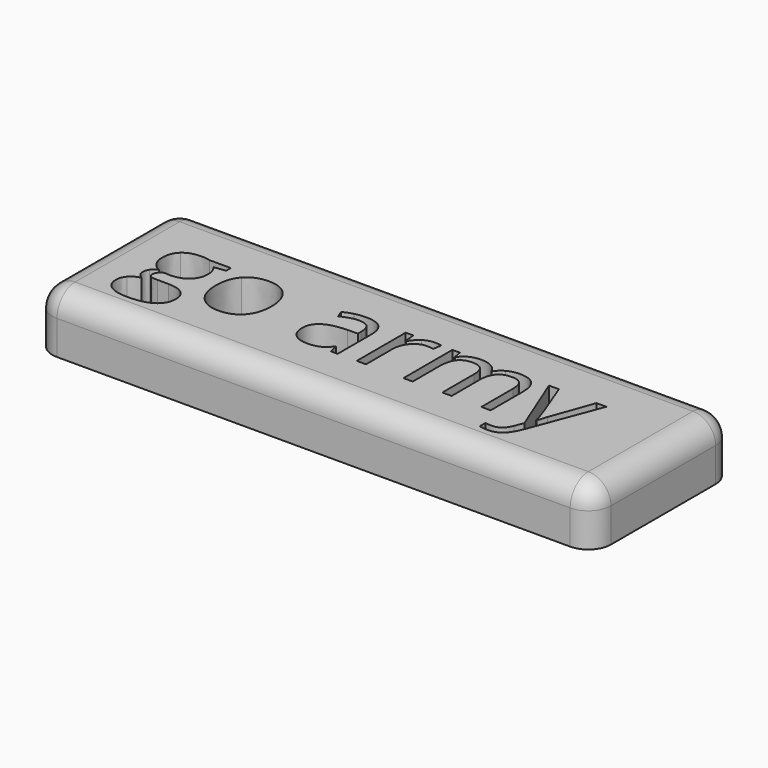
from build123d import *

# Parameters (mm, degrees)
F0_W         = 124.970305711
F0_H         = 39.4006967545
F1_DEPTH     = 12.7
F2_R         = 5.08
F3_T1_DEPTH  = 20.32
F3_S5_W      = 5.08
F3_S5_H      = 5.08
F3_T6_DEPTH  = 5.08
F3_S11_W     = 5.08
F3_S11_H     = 5.08
F3_T12_DEPTH = 5.08
F3_S17_W     = 5.08
F3_S17_H     = 5.08
F3_T18_DEPTH = 5.08
F3_S23_W     = 5.08
F3_S23_H     = 5.08
F3_T24_DEPTH = 5.08


# Not quite as in the source:
# - a fillet or chamfer that OpenCascade refuses, or shapes differently, is made with other operations: its cross-section is extruded or revolved along the edge and cut away or added


with BuildPart() as f1:
    # F0 (on Top) → F1 (new body)
    with BuildSketch(Plane.XY):
        with Locations((2.1755006164, 19.7003483772)):
            Rectangle(F0_W, F0_H)
        with BuildLine():
            Line((-42.0411116502, 26.2190565667), (-37.310148709, 26.2190565667))
            Line((-37.310148709, 26.2190565667), (-37.310148709, 24.9084519682))
            Line((-37.310148709, 24.9084519682), (-39.8434515001, 24.6087710386))
            add(Edge.make_bspline(
                [(-39.8434515001, 24.6087710386), (-39.4958216218, 24.1732347543), (-39.2201151666, 23.4659877606)],
                knots=[0, 0, 0, 1, 1, 1], degree=2))
            add(Edge.make_bspline(
                [(-39.2201151666, 23.4659877606), (-38.9444087115, 22.7587407668), (-38.9444087115, 21.8756809611)],
                knots=[0, 0, 0, 1, 1, 1], degree=2))
            add(Edge.make_bspline(
                [(-38.9444087115, 21.8756809611), (-38.9444087115, 19.8618251145), (-40.3189452417, 18.6631013963)],
                knots=[0, 0, 0, 1, 1, 1], degree=2))
            add(Edge.make_bspline(
                [(-40.3189452417, 18.6631013963), (-41.6934817719, 17.4643776781), (-44.0909292083, 17.4643776781)],
                knots=[0, 0, 0, 1, 1, 1], degree=2))
            add(Edge.make_bspline(
                [(-44.0909292083, 17.4643776781), (-44.7022783046, 17.4643776781), (-45.2377082321, 17.5642713212)],
                knots=[0, 0, 0, 1, 1, 1], degree=2))
            add(Edge.make_bspline(
                [(-45.2377082321, 17.5642713212), (-46.5603000678, 16.8650158189), (-46.5603000678, 15.8061432012)],
                knots=[0, 0, 0, 1, 1, 1], degree=2))
            add(Edge.make_bspline(
                [(-46.5603000678, 15.8061432012), (-46.5603000678, 15.2427430536), (-46.0987914363, 14.9750280899)],
                knots=[0, 0, 0, 1, 1, 1], degree=2))
            add(Edge.make_bspline(
                [(-46.0987914363, 14.9750280899), (-45.6372828048, 14.7073131262), (-44.5144782554, 14.7073131262)],
                knots=[0, 0, 0, 1, 1, 1], degree=2))
            Line((-44.5144782554, 14.7073131262), (-42.0930563446, 14.7073131262))
            add(Edge.make_bspline(
                [(-42.0930563446, 14.7073131262), (-39.8674259745, 14.7073131262), (-38.6766937477, 13.7703107531)],
                knots=[0, 0, 0, 1, 1, 1], degree=2))
            add(Edge.make_bspline(
                [(-38.6766937477, 13.7703107531), (-37.485961521, 12.83330838), (-37.485961521, 11.0472100399)],
                knots=[0, 0, 0, 1, 1, 1], degree=2))
            add(Edge.make_bspline(
                [(-37.485961521, 11.0472100399), (-37.485961521, 8.773630721), (-39.3080215727, 7.5809006214)],
                knots=[0, 0, 0, 1, 1, 1], degree=2))
            add(Edge.make_bspline(
                [(-39.3080215727, 7.5809006214), (-41.1300816243, 6.3881705218), (-44.6263591358, 6.3881705218)],
                knots=[0, 0, 0, 1, 1, 1], degree=2))
            add(Edge.make_bspline(
                [(-44.6263591358, 6.3881705218), (-47.3115002646, 6.3881705218), (-48.7659517094, 7.3871069536)],
                knots=[0, 0, 0, 1, 1, 1], degree=2))
            add(Edge.make_bspline(
                [(-48.7659517094, 7.3871069536), (-50.2204031541, 8.3860433854), (-50.2204031541, 10.2120991829)],
                knots=[0, 0, 0, 1, 1, 1], degree=2))
            add(Edge.make_bspline(
                [(-50.2204031541, 10.2120991829), (-50.2204031541, 11.4587718498), (-49.4212540086, 12.3717997485)],
                knots=[0, 0, 0, 1, 1, 1], degree=2))
            add(Edge.make_bspline(
                [(-49.4212540086, 12.3717997485), (-48.6221048632, 13.2848276472), (-47.1756449099, 13.6084830511)],
                knots=[0, 0, 0, 1, 1, 1], degree=2))
            add(Edge.make_bspline(
                [(-47.1756449099, 13.6084830511), (-47.6990876001, 13.844232049), (-48.0547089699, 14.343700265)],
                knots=[0, 0, 0, 1, 1, 1], degree=2))
            add(Edge.make_bspline(
                [(-48.0547089699, 14.343700265), (-48.4103303396, 14.8431684809), (-48.4103303396, 15.5064622716)],
                knots=[0, 0, 0, 1, 1, 1], degree=2))
            add(Edge.make_bspline(
                [(-48.4103303396, 15.5064622716), (-48.4103303396, 16.2536667227), (-48.0107557669, 16.8170668702)],
                knots=[0, 0, 0, 1, 1, 1], degree=2))
            add(Edge.make_bspline(
                [(-48.0107557669, 16.8170668702), (-47.6111811941, 17.3804670178), (-46.748100117, 17.9039097081)],
                knots=[0, 0, 0, 1, 1, 1], degree=2))
            add(Edge.make_bspline(
                [(-46.748100117, 17.9039097081), (-47.8109684805, 18.3394459923), (-48.478258017, 19.3883292458)],
                knots=[0, 0, 0, 1, 1, 1], degree=2))
            add(Edge.make_bspline(
                [(-48.478258017, 19.3883292458), (-49.1455475535, 20.4372124992), (-49.1455475535, 21.7877745551)],
                knots=[0, 0, 0, 1, 1, 1], degree=2))
            add(Edge.make_bspline(
                [(-49.1455475535, 21.7877745551), (-49.1455475535, 24.0333836539), (-47.7969833705, 25.2520861007)],
                knots=[0, 0, 0, 1, 1, 1], degree=2))
            add(Edge.make_bspline(
                [(-47.7969833705, 25.2520861007), (-46.4484191875, 26.4707885476), (-43.979048328, 26.4707885476)],
                knots=[0, 0, 0, 1, 1, 1], degree=2))
            add(Edge.make_bspline(
                [(-43.979048328, 26.4707885476), (-42.9041927273, 26.4707885476), (-42.0411116502, 26.2190565667)],
                knots=[0, 0, 0, 1, 1, 1], degree=2))
        make_face(mode=Mode.SUBTRACT)
        with BuildLine():
            add(Edge.make_bspline(
                [(-24.381913408, 24.558824217), (-22.6897150925, 22.6468598865), (-22.6897150925, 19.3903271186)],
                knots=[0, 0, 0, 1, 1, 1], degree=2))
            add(Edge.make_bspline(
                [(-22.6897150925, 19.3903271186), (-22.6897150925, 16.0418921991), (-24.3739219166, 14.1618938344)],
                knots=[0, 0, 0, 1, 1, 1], degree=2))
            add(Edge.make_bspline(
                [(-24.3739219166, 14.1618938344), (-26.0581287407, 12.2818954696), (-29.0309635618, 12.2818954696)],
                knots=[0, 0, 0, 1, 1, 1], degree=2))
            add(Edge.make_bspline(
                [(-29.0309635618, 12.2818954696), (-30.8690065964, 12.2818954696), (-32.2914920754, 13.1449765468)],
                knots=[0, 0, 0, 1, 1, 1], degree=2))
            add(Edge.make_bspline(
                [(-32.2914920754, 13.1449765468), (-33.7139775543, 14.0080576239), (-34.4891522254, 15.618343152)],
                knots=[0, 0, 0, 1, 1, 1], degree=2))
            add(Edge.make_bspline(
                [(-34.4891522254, 15.618343152), (-35.2643268965, 17.2286286801), (-35.2643268965, 19.3903271186)],
                knots=[0, 0, 0, 1, 1, 1], degree=2))
            add(Edge.make_bspline(
                [(-35.2643268965, 19.3903271186), (-35.2643268965, 22.7347662925), (-33.5901094368, 24.60277742)],
                knots=[0, 0, 0, 1, 1, 1], degree=2))
            add(Edge.make_bspline(
                [(-33.5901094368, 24.60277742), (-31.915891977, 26.4707885476), (-28.9430571558, 26.4707885476)],
                knots=[0, 0, 0, 1, 1, 1], degree=2))
            add(Edge.make_bspline(
                [(-28.9430571558, 26.4707885476), (-26.0741117236, 26.4707885476), (-24.381913408, 24.558824217)],
                knots=[0, 0, 0, 1, 1, 1], degree=2))
        make_face(mode=Mode.SUBTRACT)
        with BuildLine():
            Line((-2.455258729, 12.5336274505), (-3.9936208341, 12.5336274505))
            Line((-3.9936208341, 12.5336274505), (-4.405182644, 14.4835513654))
            Line((-4.405182644, 14.4835513654), (-4.5050762872, 14.4835513654))
            add(Edge.make_bspline(
                [(-4.5050762872, 14.4835513654), (-5.5279871934, 13.1969212412), (-6.544904481, 12.7394083554)],
                knots=[0, 0, 0, 1, 1, 1], degree=2))
            add(Edge.make_bspline(
                [(-6.544904481, 12.7394083554), (-7.5618217686, 12.2818954696), (-9.0881966365, 12.2818954696)],
                knots=[0, 0, 0, 1, 1, 1], degree=2))
            add(Edge.make_bspline(
                [(-9.0881966365, 12.2818954696), (-11.1220312117, 12.2818954696), (-12.2768017269, 13.3327765959)],
                knots=[0, 0, 0, 1, 1, 1], degree=2))
            add(Edge.make_bspline(
                [(-12.2768017269, 13.3327765959), (-13.4315722421, 14.3836577222), (-13.4315722421, 16.3175986543)],
                knots=[0, 0, 0, 1, 1, 1], degree=2))
            add(Edge.make_bspline(
                [(-13.4315722421, 16.3175986543), (-13.4315722421, 20.4611869736), (-6.8026300804, 20.66097426)],
                knots=[0, 0, 0, 1, 1, 1], degree=2))
            Line((-6.8026300804, 20.66097426), (-4.4811018128, 20.7368934288))
            Line((-4.4811018128, 20.7368934288), (-4.4811018128, 21.5879872687))
            add(Edge.make_bspline(
                [(-4.4811018128, 21.5879872687), (-4.4811018128, 23.1982727968), (-5.1723658237, 23.9654559765)],
                knots=[0, 0, 0, 1, 1, 1], degree=2))
            add(Edge.make_bspline(
                [(-5.1723658237, 23.9654559765), (-5.8636298345, 24.7326391562), (-7.3900047024, 24.7326391562)],
                knots=[0, 0, 0, 1, 1, 1], degree=2))
            add(Edge.make_bspline(
                [(-7.3900047024, 24.7326391562), (-9.1001838737, 24.7326391562), (-11.2578865665, 23.6857537756)],
                knots=[0, 0, 0, 1, 1, 1], degree=2))
            Line((-11.2578865665, 23.6857537756), (-11.8972058828, 25.2720648293))
            add(Edge.make_bspline(
                [(-11.8972058828, 25.2720648293), (-10.8862822138, 25.819481994), (-9.681564877, 26.1311501607)],
                knots=[0, 0, 0, 1, 1, 1], degree=2))
            add(Edge.make_bspline(
                [(-9.681564877, 26.1311501607), (-8.4768475402, 26.4428183275), (-7.2621408391, 26.4428183275)],
                knots=[0, 0, 0, 1, 1, 1], degree=2))
            add(Edge.make_bspline(
                [(-7.2621408391, 26.4428183275), (-4.8167444539, 26.4428183275), (-3.6360015915, 25.3579733625)],
                knots=[0, 0, 0, 1, 1, 1], degree=2))
            add(Edge.make_bspline(
                [(-3.6360015915, 25.3579733625), (-2.455258729, 24.2731283975), (-2.455258729, 21.8756809611)],
                knots=[0, 0, 0, 1, 1, 1], degree=2))
            Line((-2.455258729, 21.8756809611), (-2.455258729, 12.5336274505))
        make_face(mode=Mode.SUBTRACT)
        with BuildLine():
            add(Edge.make_bspline(
                [(5.6960625548, 25.745560698), (6.7709181555, 26.4707885476), (8.0575482797, 26.4707885476)],
                knots=[0, 0, 0, 1, 1, 1], degree=2))
            add(Edge.make_bspline(
                [(8.0575482797, 26.4707885476), (8.9685783055, 26.4707885476), (9.6918082822, 26.3189502099)],
                knots=[0, 0, 0, 1, 1, 1], degree=2))
            Line((9.6918082822, 26.3189502099), (9.4041145898, 24.3969965151))
            add(Edge.make_bspline(
                [(9.4041145898, 24.3969965151), (8.5570164956, 24.5847965642), (7.9057099421, 24.5847965642)],
                knots=[0, 0, 0, 1, 1, 1], degree=2))
            add(Edge.make_bspline(
                [(7.9057099421, 24.5847965642), (6.2434797195, 24.5847965642), (5.0647347299, 23.2362323812)],
                knots=[0, 0, 0, 1, 1, 1], degree=2))
            add(Edge.make_bspline(
                [(5.0647347299, 23.2362323812), (3.8859897403, 21.8876681983), (3.8859897403, 19.8778080974)],
                knots=[0, 0, 0, 1, 1, 1], degree=2))
            Line((3.8859897403, 19.8778080974), (3.8859897403, 12.5336274505))
            Line((3.8859897403, 12.5336274505), (1.8121977078, 12.5336274505))
            Line((1.8121977078, 12.5336274505), (1.8121977078, 26.2190565667))
            Line((1.8121977078, 26.2190565667), (3.5223768791, 26.2190565667))
            Line((3.5223768791, 26.2190565667), (3.7621216228, 23.6857537756))
            Line((3.7621216228, 23.6857537756), (3.8620152659, 23.6857537756))
            add(Edge.make_bspline(
                [(3.8620152659, 23.6857537756), (4.6212069541, 25.0203328485), (5.6960625548, 25.745560698)],
                knots=[0, 0, 0, 1, 1, 1], degree=2))
        make_face(mode=Mode.SUBTRACT)
        with BuildLine():
            Line((31.768303426, 12.5336274505), (29.6985071392, 12.5336274505))
            Line((29.6985071392, 12.5336274505), (29.6985071392, 21.4361489311))
            add(Edge.make_bspline(
                [(29.6985071392, 21.4361489311), (29.6985071392, 23.0744046793), (28.9992516369, 23.8915346805)],
                knots=[0, 0, 0, 1, 1, 1], degree=2))
            add(Edge.make_bspline(
                [(28.9992516369, 23.8915346805), (28.2999961346, 24.7086646818), (26.8255659612, 24.7086646818)],
                knots=[0, 0, 0, 1, 1, 1], degree=2))
            add(Edge.make_bspline(
                [(26.8255659612, 24.7086646818), (24.8916250291, 24.7086646818), (23.9666098933, 23.5978473696)],
                knots=[0, 0, 0, 1, 1, 1], degree=2))
            add(Edge.make_bspline(
                [(23.9666098933, 23.5978473696), (23.0415947574, 22.4870300574), (23.0415947574, 20.1774890269)],
                knots=[0, 0, 0, 1, 1, 1], degree=2))
            Line((23.0415947574, 20.1774890269), (23.0415947574, 12.5336274505))
            Line((23.0415947574, 12.5336274505), (20.9678027249, 12.5336274505))
            Line((20.9678027249, 12.5336274505), (20.9678027249, 21.4361489311))
            add(Edge.make_bspline(
                [(20.9678027249, 21.4361489311), (20.9678027249, 23.0744046793), (20.2685472226, 23.8915346805)],
                knots=[0, 0, 0, 1, 1, 1], degree=2))
            add(Edge.make_bspline(
                [(20.2685472226, 23.8915346805), (19.5692917203, 24.7086646818), (18.0828743097, 24.7086646818)],
                knots=[0, 0, 0, 1, 1, 1], degree=2))
            add(Edge.make_bspline(
                [(18.0828743097, 24.7086646818), (16.1369461405, 24.7086646818), (15.2319097332, 23.5419069294)],
                knots=[0, 0, 0, 1, 1, 1], degree=2))
            add(Edge.make_bspline(
                [(15.2319097332, 23.5419069294), (14.3268733259, 22.375149177), (14.3268733259, 19.7139825226)],
                knots=[0, 0, 0, 1, 1, 1], degree=2))
            Line((14.3268733259, 19.7139825226), (14.3268733259, 12.5336274505))
            Line((14.3268733259, 12.5336274505), (12.2530812934, 12.5336274505))
            Line((12.2530812934, 12.5336274505), (12.2530812934, 26.2190565667))
            Line((12.2530812934, 26.2190565667), (13.9392859904, 26.2190565667))
            Line((13.9392859904, 26.2190565667), (14.2749286315, 24.3450518206))
            Line((14.2749286315, 24.3450518206), (14.3748222747, 24.3450518206))
            add(Edge.make_bspline(
                [(14.3748222747, 24.3450518206), (14.9621968966, 25.3439882524), (16.0310588787, 25.9073884)],
                knots=[0, 0, 0, 1, 1, 1], degree=2))
            add(Edge.make_bspline(
                [(16.0310588787, 25.9073884), (17.0999208608, 26.4707885476), (18.4225126965, 26.4707885476)],
                knots=[0, 0, 0, 1, 1, 1], degree=2))
            add(Edge.make_bspline(
                [(18.4225126965, 26.4707885476), (21.6310965156, 26.4707885476), (22.6180457103, 24.1452645342)],
                knots=[0, 0, 0, 1, 1, 1], degree=2))
            Line((22.6180457103, 24.1452645342), (22.7179393534, 24.1452645342))
            add(Edge.make_bspline(
                [(22.7179393534, 24.1452645342), (23.3292884497, 25.2201201349), (24.4900525835, 25.8454543412)],
                knots=[0, 0, 0, 1, 1, 1], degree=2))
            add(Edge.make_bspline(
                [(24.4900525835, 25.8454543412), (25.6508167173, 26.4707885476), (27.1372341279, 26.4707885476)],
                knots=[0, 0, 0, 1, 1, 1], degree=2))
            add(Edge.make_bspline(
                [(27.1372341279, 26.4707885476), (29.4587623955, 26.4707885476), (30.6135329107, 25.2780584479)],
                knots=[0, 0, 0, 1, 1, 1], degree=2))
            add(Edge.make_bspline(
                [(30.6135329107, 25.2780584479), (31.768303426, 24.0853283483), (31.768303426, 21.4601234054)],
                knots=[0, 0, 0, 1, 1, 1], degree=2))
            Line((31.768303426, 21.4601234054), (31.768303426, 12.5336274505))
        make_face(mode=Mode.SUBTRACT)
        with BuildLine():
            Line((39.3881905281, 12.4577082816), (33.8660699328, 26.2190565667))
            Line((33.8660699328, 26.2190565667), (36.091700303, 26.2190565667))
            Line((36.091700303, 26.2190565667), (39.0885095985, 18.4153651612))
            add(Edge.make_bspline(
                [(39.0885095985, 18.4153651612), (40.0714630474, 15.7422112696), (40.3112077911, 14.5554747885)],
                knots=[0, 0, 0, 1, 1, 1], degree=2))
            Line((40.3112077911, 14.5554747885), (40.4111014343, 14.5554747885))
            add(Edge.make_bspline(
                [(40.4111014343, 14.5554747885), (40.5709312634, 15.1947941049), (41.0903782079, 16.7371519557)],
                knots=[0, 0, 0, 1, 1, 1], degree=2))
            add(Edge.make_bspline(
                [(41.0903782079, 16.7371519557), (41.6098251525, 18.2795098064), (44.4827663305, 26.2190565667)],
                knots=[0, 0, 0, 1, 1, 1], degree=2))
            Line((44.4827663305, 26.2190565667), (46.7044009549, 26.2190565667))
            Line((46.7044009549, 26.2190565667), (40.8226632442, 10.63564823))
            add(Edge.make_bspline(
                [(40.8226632442, 10.63564823), (39.9475949299, 8.3261071995), (38.7808371775, 7.3571388606)],
                knots=[0, 0, 0, 1, 1, 1], degree=2))
            add(Edge.make_bspline(
                [(38.7808371775, 7.3571388606), (37.6140794251, 6.3881705218), (35.915887491, 6.3881705218)],
                knots=[0, 0, 0, 1, 1, 1], degree=2))
            add(Edge.make_bspline(
                [(35.915887491, 6.3881705218), (34.9649000079, 6.3881705218), (34.0418827448, 6.603940791)],
                knots=[0, 0, 0, 1, 1, 1], degree=2))
            Line((34.0418827448, 6.603940791), (34.0418827448, 8.2621752679))
            add(Edge.make_bspline(
                [(34.0418827448, 8.2621752679), (34.7291510099, 8.114332676), (35.5762491041, 8.114332676)],
                knots=[0, 0, 0, 1, 1, 1], degree=2))
            add(Edge.make_bspline(
                [(35.5762491041, 8.114332676), (37.7139730683, 8.114332676), (38.6250030941, 10.5117801124)],
                knots=[0, 0, 0, 1, 1, 1], degree=2))
            Line((38.6250030941, 10.5117801124), (39.3881905281, 12.4577082816))
        make_face(mode=Mode.SUBTRACT)
    extrude(amount=F1_DEPTH)

    # F2
    f2_edges = [f1.edges().sort_by_distance(p)[0] for p in [
        (2.175501, 39.400697, 12.7),
        (-60.309652, 19.700348, 12.7),
        (64.660653, 19.700348, 12.7),
        (2.175501, 0, 12.7),
    ]]
    fillet(f2_edges, radius=F2_R)

    # F3: fillet of radius 5.08 on 4 edges, made by hand

    # F3_s2 → F3_t1 (cut)
    with BuildSketch(Plane.XY.offset(-12.7)):
        with BuildLine():
            ThreePointArc((64.6606534719, 5.08), (63.1727559204, 1.4878975516), (59.5806534719, 0))
            Line((59.5806534719, 0), (64.6606534719, 0))
            Line((64.6606534719, 0), (64.6606534719, 5.08))
        make_face()
        with BuildLine():
            ThreePointArc((-60.3096522391, 5.08), (-58.8217546875, 1.4878975516), (-55.2296522391, 0))
            Line((-55.2296522391, 0), (-60.3096522391, 0))
            Line((-60.3096522391, 0), (-60.3096522391, 5.08))
        make_face()
        with BuildLine():
            ThreePointArc((-55.2296522391, 39.4006967545), (-58.8217546875, 37.9127992029), (-60.3096522391, 34.3206967545))
            Line((-60.3096522391, 34.3206967545), (-60.3096522391, 39.4006967545))
            Line((-60.3096522391, 39.4006967545), (-55.2296522391, 39.4006967545))
        make_face()
        with BuildLine():
            ThreePointArc((59.5806534719, 39.4006967545), (63.1727559204, 37.9127992029), (64.6606534719, 34.3206967545))
            Line((64.6606534719, 34.3206967545), (64.6606534719, 39.4006967545))
            Line((64.6606534719, 39.4006967545), (59.5806534719, 39.4006967545))
        make_face()
    extrude(amount=F3_T1_DEPTH, mode=Mode.SUBTRACT)


with BuildPart() as f3_tool4:
    # F3_s5 → F3_t6 (new body)
    with BuildSketch(Plane.XZ.offset(-34.3206967545)):
        with Locations((62.1206534719, 10.16)):
            Rectangle(F3_S5_W, F3_S5_H)
    extrude(amount=-F3_T6_DEPTH)

    # F3_s7 → F3_t8 (revolve, cut)
    with BuildSketch(Plane(origin=(59.5806534719, 34.3206967545, 7.62), x_dir=(-0.7071067812, 0, -0.7071067812), z_dir=(0.7071067812, 0, -0.7071067812))):
        with BuildLine():
            ThreePointArc((0, -5.08), (5.08, 0), (0, 5.08))
            Line((0, 5.08), (0, -5.08))
        make_face()
    revolve(axis=Axis((59.5806534719, 34.3206967545, 7.62), (0, 1, 0)), mode=Mode.SUBTRACT)


with BuildPart() as f1_1:
    add(f1.part)

    # F3_t3: cut F3_tool4
    add(f3_tool4.part, mode=Mode.SUBTRACT)


with BuildPart() as f3_tool10:
    # F3_s11 → F3_t12 (new body)
    with BuildSketch(Plane.XZ.offset(-34.3206967545)):
        with Locations((-57.7696522391, 10.16)):
            Rectangle(F3_S11_W, F3_S11_H)
    extrude(amount=-F3_T12_DEPTH)

    # F3_s13 → F3_t14 (revolve, cut)
    with BuildSketch(Plane(origin=(-55.2296522391, 34.3206967545, 7.62), x_dir=(0.7071067812, 0, -0.7071067812), z_dir=(0.7071067812, 0, 0.7071067812))):
        with BuildLine():
            ThreePointArc((0, -5.08), (5.08, 0), (0, 5.08))
            Line((0, 5.08), (0, -5.08))
        make_face()
    revolve(axis=Axis((-55.2296522391, 34.3206967545, 7.62), (0, 1, 0)), mode=Mode.SUBTRACT)


with BuildPart() as f1_2:
    add(f1_1.part)

    # F3_t9: cut F3_tool10
    add(f3_tool10.part, mode=Mode.SUBTRACT)


with BuildPart() as f3_tool16:
    # F3_s17 → F3_t18 (new body)
    with BuildSketch(Plane.YZ.offset(-55.2296522391)):
        with Locations((2.54, 10.16)):
            Rectangle(F3_S17_W, F3_S17_H)
    extrude(amount=-F3_T18_DEPTH)

    # F3_s19 → F3_t20 (revolve, cut)
    with BuildSketch(Plane(origin=(-55.2296522391, 5.08, 7.62), x_dir=(0, 0.7071067812, -0.7071067812), z_dir=(0, 0.7071067812, 0.7071067812))):
        with BuildLine():
            ThreePointArc((0, -5.08), (5.08, 0), (0, 5.08))
            Line((0, 5.08), (0, -5.08))
        make_face()
    revolve(axis=Axis((-55.2296522391, 5.08, 7.62), (-1, 0, 0)), mode=Mode.SUBTRACT)


with BuildPart() as f1_3:
    add(f1_2.part)

    # F3_t15: cut F3_tool16
    add(f3_tool16.part, mode=Mode.SUBTRACT)


with BuildPart() as f3_tool22:
    # F3_s23 → F3_t24 (new body)
    with BuildSketch(Plane.YZ.offset(59.5806534719)):
        with Locations((2.54, 10.16)):
            Rectangle(F3_S23_W, F3_S23_H)
    extrude(amount=F3_T24_DEPTH)

    # F3_s25 → F3_t26 (revolve, cut)
    with BuildSketch(Plane(origin=(59.5806534719, 5.08, 7.62), x_dir=(0, 0.7071067812, -0.7071067812), z_dir=(0, -0.7071067812, -0.7071067812))):
        with BuildLine():
            ThreePointArc((0, -5.08), (5.08, 0), (0, 5.08))
            Line((0, 5.08), (0, -5.08))
        make_face()
    revolve(axis=Axis((59.5806534719, 5.08, 7.62), (1, 0, 0)), mode=Mode.SUBTRACT)


with BuildPart() as f1_4:
    add(f1_3.part)

    # F3_t21: cut F3_tool22
    add(f3_tool22.part, mode=Mode.SUBTRACT)


solid = f1_4.part
